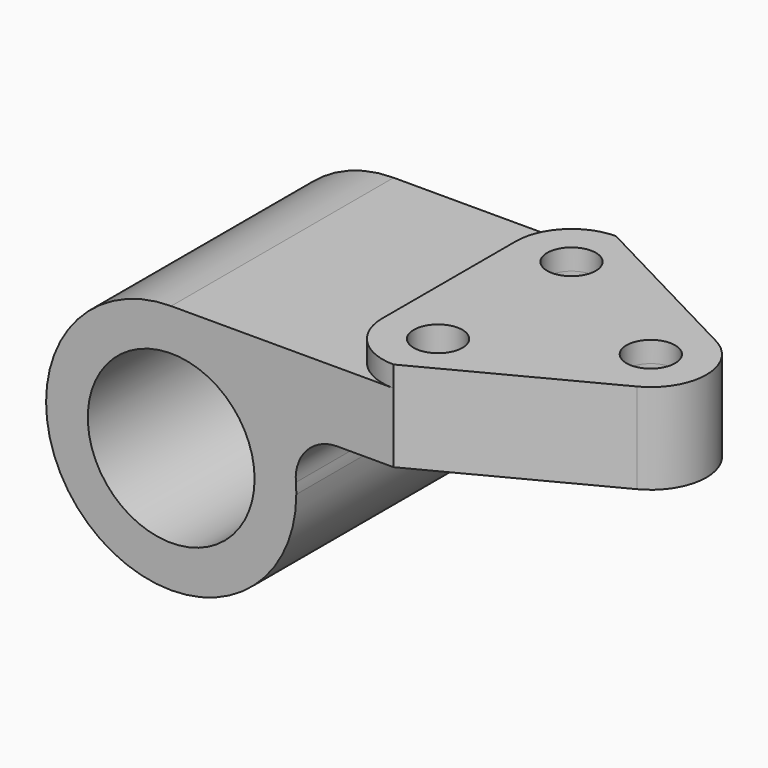
from build123d import *

# Parameters (mm, degrees)
F0_R          = 19.05
F1_DEPTH      = 63.5
F2_R          = 5.5626
F3_DEPTH      = 4.7752
F3_DEPTH_BACK = 15.875
F4_DEPTH      = 57.151


with BuildPart() as f1:
    # F0 (on Front) → F1 (new body)
    with BuildSketch(Plane.XZ):
        with BuildLine():
            ThreePointArc((0, 28.575), (19.345366451, 21.0306305629), (28.4756083945, 2.38125))
            ThreePointArc((28.4756083945, 2.38125), (30.9572676717, 9.6234554837), (37.9674778593, 12.7))
            Line((37.9674778593, 12.7), (50.8, 12.7))
            Line((50.8, 12.7), (50.8, 28.575))
            Line((50.8, 28.575), (0, 28.575))
        make_face()
        with BuildLine():
            ThreePointArc((0, 28.575), (-20.2055762724, -20.2055762724), (28.575, 0))
            ThreePointArc((28.575, 0), (28.5501412858, 1.1916616816), (28.4756083945, 2.38125))
            ThreePointArc((28.4756083945, 2.38125), (19.345366451, 21.0306305629), (0, 28.575))
        make_face()
        Circle(F0_R, mode=Mode.SUBTRACT)
    extrude(amount=F1_DEPTH)

    # F2 (on face) → F3 (join, two sides)
    with BuildSketch(Plane.XY.offset(28.575)) as f3_sk:
        with BuildLine():
            Line((90.0304863666, -20.4933472006), (50.8, 0))
            ThreePointArc((50.8, 0), (41.8197438789, -3.7197438789), (38.1, -12.7))
            Line((38.1, -12.7), (38.1, -50.8))
            ThreePointArc((38.1, -50.8), (41.8197438789, -59.7802561211), (50.8, -63.5))
            Line((50.8, -63.5), (90.0304863666, -43.0066527994))
            ThreePointArc((90.0304863666, -43.0066527994), (96.8502, -31.75), (90.0304863666, -20.4933472006))
        make_face()
        with Locations((50.8, -50.8)):
            Circle(F2_R, mode=Mode.SUBTRACT)
        with Locations((50.8, -12.7)):
            Circle(F2_R, mode=Mode.SUBTRACT)
        with Locations((84.1502, -31.75)):
            Circle(F2_R, mode=Mode.SUBTRACT)
    extrude(amount=F3_DEPTH)
    extrude(f3_sk.sketch, amount=-F3_DEPTH_BACK)

    # F2 (on face) → F4 (cut, through all)
    with BuildSketch(Plane.XY.offset(28.575)):
        with BuildLine():
            Line((50.8, -18.2626), (50.8, -7.1374))
            ThreePointArc((50.8, -7.1374), (45.2374, -12.7), (50.8, -18.2626))
        make_face()
        with BuildLine():
            Line((50.8, -56.3626), (50.8, -45.2374))
            ThreePointArc((50.8, -45.2374), (45.2374, -50.8), (50.8, -56.3626))
        make_face()
    extrude(amount=-F4_DEPTH, mode=Mode.SUBTRACT)


solid = f1.part
